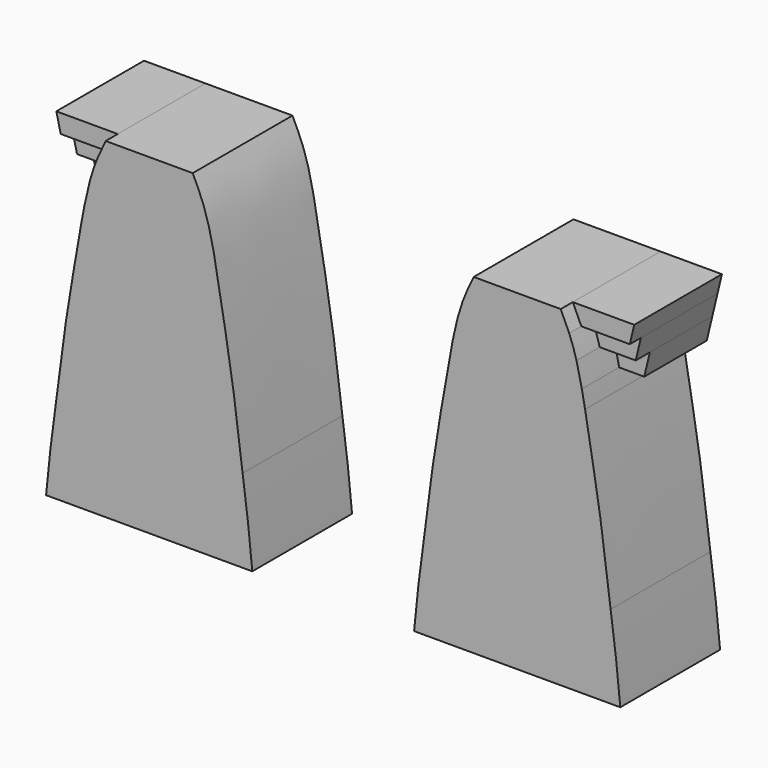
from build123d import *

# Parameters (mm, degrees)
F1_DEPTH = 25.146
F2_DEPTH = 22.098
F3_DEPTH = 19.304
F4_DEPTH = 15.748


# Not quite as in the source:
# - a feature names something its author has since deleted; it is built from what else it names


with BuildPart() as f1:
    # F0 (on Front) → F1 (new body)
    with BuildSketch(Plane.XZ):
        with BuildLine():
            add(Edge.make_bspline(
                [(18.2603467256, -50.0062517822), (18.9200009821, -44.7411017766), (20.2069897283, -34.4687678414), (22.6027171981, -20.9673750462), (24.964728506, -6.9558000416), (27.3280893956, -2.0652493334), (28.3261220902, 0)],
                knots=[0, 0, 0, 0, 0.2787145144, 0.5437734084, 0.8073383305, 1, 1, 1, 1], degree=3))
            add(Edge.make_bspline(
                [(18.2603467256, -50.0062517822), (17.8821318051, -52.7888494967), (17.1179839852, -58.354700738), (16.5830328982, -64.0164932483), (16.3121369904, -66.782541573)],
                knots=[0, 0, 0, 0, 0.4998751742, 1, 1, 1, 1], degree=3))
            Line((16.3121369904, -66.782541573), (37.1014112607, -66.782541573))
            Line((37.1014112607, -66.782541573), (57.890685531, -66.782541573))
            add(Edge.make_bspline(
                [(55.9424757957, -50.0062517822), (56.3206907163, -52.7888494967), (57.0848385361, -58.354700738), (57.6197896231, -64.0164932483), (57.890685531, -66.782541573)],
                knots=[0, 0, 0, 0, 0.4998751742, 1, 1, 1, 1], degree=3))
            add(Edge.make_bspline(
                [(55.9424757957, -50.0062517822), (55.2828215393, -44.7411017766), (53.995832793, -34.4687678414), (52.1449488151, -24.0379020943), (51.0519382112, -17.6595205046), (50.787943229, -16.1955729126)],
                knots=[0, 0, 0, 0, 0.2787145144, 0.5437734084, 0.6237310377, 0.6237310377, 0.6237310377, 0.6237310377], degree=3))
            add(Edge.make_bspline(
                [(50.787943229, -16.1955729126), (50.5801603578, -15.0433417924), (50.3657554699, -13.8999341074), (50.1413285617, -12.7882305847)],
                knots=[0.6237310377, 0.6237310377, 0.6237310377, 0.6237310377, 0.6866633921, 0.6866633921, 0.6866633921, 0.6866633921], degree=3))
            add(Edge.make_bspline(
                [(50.1413285617, -12.7882305847), (49.8063148795, -11.1287330959), (49.4489690484, -9.5398822483), (49.0579815986, -8.0977864563)],
                knots=[0.6866633921, 0.6866633921, 0.6866633921, 0.6866633921, 0.7806057805, 0.7806057805, 0.7806057805, 0.7806057805], degree=3))
            add(Edge.make_bspline(
                [(49.0579815986, -8.0977864563), (48.9467209446, -7.6874190111), (48.4886567249, -6.0860553408), (47.9823899415, -4.7049290916), (47.5862966388, -3.7397006431)],
                knots=[0.7806057805, 0.7806057805, 0.7806057805, 0.7806057805, 0.8073383305, 0.8880343317, 0.8880343317, 0.8880343317, 0.8880343317], degree=3))
            add(Edge.make_bspline(
                [(47.5862966388, -3.7397006431), (47.0367173451, -2.4004465697), (46.4567088881, -1.2002232848), (45.8767004311, 0)],
                knots=[0.8880343317, 0.8880343317, 0.8880343317, 0.8880343317, 1, 1, 1, 1], degree=3))
            Line((45.8767004311, 0), (28.3261220902, 0))
        make_face()
    extrude(amount=F1_DEPTH)


with BuildPart() as f1b:
    # F0 (on Front) → F1, piece 2 (new body)
    with BuildSketch(Plane.XZ):
        with BuildLine():
            add(Edge.make_bspline(
                [(-55.9424757957, -50.0062517822), (-55.2828215393, -44.7411017766), (-53.995832793, -34.4687678414), (-52.1449488151, -24.0379020943), (-51.0519382112, -17.6595205046), (-50.787943229, -16.1955729126)],
                knots=[0, 0, 0, 0, 0.2787145144, 0.5437734084, 0.6237310377, 0.6237310377, 0.6237310377, 0.6237310377], degree=3))
            add(Edge.make_bspline(
                [(-55.9424757957, -50.0062517822), (-56.3206907163, -52.7888494967), (-57.0848385361, -58.354700738), (-57.6197896231, -64.0164932483), (-57.890685531, -66.782541573)],
                knots=[0, 0, 0, 0, 0.4998751742, 1, 1, 1, 1], degree=3))
            Line((-57.890685531, -66.782541573), (-37.1014112607, -66.782541573))
            Line((-37.1014112607, -66.782541573), (-16.3121369904, -66.782541573))
            add(Edge.make_bspline(
                [(-18.2603467256, -50.0062517822), (-17.8821318051, -52.7888494967), (-17.1179839852, -58.354700738), (-16.5830328982, -64.0164932483), (-16.3121369904, -66.782541573)],
                knots=[0, 0, 0, 0, 0.4998751742, 1, 1, 1, 1], degree=3))
            add(Edge.make_bspline(
                [(-18.2603467256, -50.0062517822), (-18.9200009821, -44.7411017766), (-20.2069897283, -34.4687678414), (-22.6027171981, -20.9673750462), (-24.964728506, -6.9558000416), (-27.3280893956, -2.0652493334), (-28.3261220902, 0)],
                knots=[0, 0, 0, 0, 0.2787145144, 0.5437734084, 0.8073383305, 1, 1, 1, 1], degree=3))
            Line((-28.3261220902, 0), (-45.8767004311, 0))
            add(Edge.make_bspline(
                [(-47.5862966388, -3.7397006431), (-47.0367173451, -2.4004465697), (-46.4567088881, -1.2002232848), (-45.8767004311, 0)],
                knots=[0.8880343317, 0.8880343317, 0.8880343317, 0.8880343317, 1, 1, 1, 1], degree=3))
            add(Edge.make_bspline(
                [(-49.0579815986, -8.0977864563), (-48.9467209446, -7.6874190111), (-48.4886567249, -6.0860553408), (-47.9823899415, -4.7049290916), (-47.5862966388, -3.7397006431)],
                knots=[0.7806057805, 0.7806057805, 0.7806057805, 0.7806057805, 0.8073383305, 0.8880343317, 0.8880343317, 0.8880343317, 0.8880343317], degree=3))
            add(Edge.make_bspline(
                [(-50.1413285617, -12.7882305847), (-49.8063148795, -11.1287330959), (-49.4489690484, -9.5398822483), (-49.0579815986, -8.0977864563)],
                knots=[0.6866633921, 0.6866633921, 0.6866633921, 0.6866633921, 0.7806057805, 0.7806057805, 0.7806057805, 0.7806057805], degree=3))
            add(Edge.make_bspline(
                [(-50.787943229, -16.1955729126), (-50.5801603578, -15.0433417924), (-50.3657554699, -13.8999341074), (-50.1413285617, -12.7882305847)],
                knots=[0.6237310377, 0.6237310377, 0.6237310377, 0.6237310377, 0.6866633921, 0.6866633921, 0.6866633921, 0.6866633921], degree=3))
        make_face()
    extrude(amount=F1_DEPTH)


with BuildPart() as f2:
    # F0 (on Front) → F2 (new body)
    with BuildSketch(Plane.XZ):
        with BuildLine():
            Line((58.2653470337, 0), (45.8767004311, 0))
            add(Edge.make_bspline(
                [(47.5862966388, -3.7397006431), (47.0367173451, -2.4004465697), (46.4567088881, -1.2002232848), (45.8767004311, 0)],
                knots=[0.8880343317, 0.8880343317, 0.8880343317, 0.8880343317, 1, 1, 1, 1], degree=3))
            Line((47.5862966388, -3.7397006431), (57.3713946033, -3.7397006431))
            Line((57.3713946033, -3.7397006431), (58.2653470337, 0))
        make_face()
    extrude(amount=F2_DEPTH)


with BuildPart() as f2b:
    # F0 (on Front) → F2, piece 2 (new body)
    with BuildSketch(Plane.XZ):
        with BuildLine():
            Line((-57.3713946033, -3.7397006431), (-47.5862966388, -3.7397006431))
            add(Edge.make_bspline(
                [(-47.5862966388, -3.7397006431), (-47.0367173451, -2.4004465697), (-46.4567088881, -1.2002232848), (-45.8767004311, 0)],
                knots=[0.8880343317, 0.8880343317, 0.8880343317, 0.8880343317, 1, 1, 1, 1], degree=3))
            Line((-45.8767004311, 0), (-58.2653470337, 0))
            Line((-58.2653470337, 0), (-57.3713946033, -3.7397006431))
        make_face()
    extrude(amount=F2_DEPTH)


with BuildPart() as f3:
    # F0 (on Front) → F3 (new body)
    with BuildSketch(Plane.XZ):
        with BuildLine():
            Line((57.3713946033, -3.7397006431), (47.5862966388, -3.7397006431))
            add(Edge.make_bspline(
                [(49.0579815986, -8.0977864563), (48.9467209446, -7.6874190111), (48.4886567249, -6.0860553408), (47.9823899415, -4.7049290916), (47.5862966388, -3.7397006431)],
                knots=[0.7806057805, 0.7806057805, 0.7806057805, 0.7806057805, 0.8073383305, 0.8880343317, 0.8880343317, 0.8880343317, 0.8880343317], degree=3))
            Line((49.0579815986, -8.0977864563), (56.3296210025, -8.0977864563))
            Line((56.3296210025, -8.0977864563), (57.3713946033, -3.7397006431))
        make_face()
    extrude(amount=F3_DEPTH)


with BuildPart() as f3b:
    # F0 (on Front) → F3, piece 2 (new body)
    with BuildSketch(Plane.XZ):
        with BuildLine():
            Line((-56.3296210025, -8.0977864563), (-49.0579815986, -8.0977864563))
            add(Edge.make_bspline(
                [(-49.0579815986, -8.0977864563), (-48.9467209446, -7.6874190111), (-48.4886567249, -6.0860553408), (-47.9823899415, -4.7049290916), (-47.5862966388, -3.7397006431)],
                knots=[0.7806057805, 0.7806057805, 0.7806057805, 0.7806057805, 0.8073383305, 0.8880343317, 0.8880343317, 0.8880343317, 0.8880343317], degree=3))
            Line((-47.5862966388, -3.7397006431), (-57.3713946033, -3.7397006431))
            Line((-57.3713946033, -3.7397006431), (-56.3296210025, -8.0977864563))
        make_face()
    extrude(amount=F3_DEPTH)


with BuildPart() as f4:
    # F0 (on Front) → F4 (new body)
    with BuildSketch(Plane.XZ):
        with BuildLine():
            Line((-55.2083991912, -12.7882305847), (-50.1413285617, -12.7882305847))
            add(Edge.make_bspline(
                [(-50.1413285617, -12.7882305847), (-49.8063148795, -11.1287330959), (-49.4489690484, -9.5398822483), (-49.0579815986, -8.0977864563)],
                knots=[0.6866633921, 0.6866633921, 0.6866633921, 0.6866633921, 0.7806057805, 0.7806057805, 0.7806057805, 0.7806057805], degree=3))
            Line((-49.0579815986, -8.0977864563), (-56.3296210025, -8.0977864563))
            Line((-56.3296210025, -8.0977864563), (-55.2083991912, -12.7882305847))
        make_face()
    extrude(amount=F4_DEPTH)


with BuildPart() as f4b:
    # F0 (on Front) → F4, piece 2 (new body)
    with BuildSketch(Plane.XZ):
        with BuildLine():
            Line((56.3296210025, -8.0977864563), (49.0579815986, -8.0977864563))
            add(Edge.make_bspline(
                [(50.1413285617, -12.7882305847), (49.8063148795, -11.1287330959), (49.4489690484, -9.5398822483), (49.0579815986, -8.0977864563)],
                knots=[0.6866633921, 0.6866633921, 0.6866633921, 0.6866633921, 0.7806057805, 0.7806057805, 0.7806057805, 0.7806057805], degree=3))
            Line((50.1413285617, -12.7882305847), (55.2083991912, -12.7882305847))
            Line((55.2083991912, -12.7882305847), (56.3296210025, -8.0977864563))
        make_face()
    extrude(amount=F4_DEPTH)


solid = Compound([f1.part, f1b.part, f2.part, f2b.part, f3.part, f3b.part, f4.part, f4b.part])
